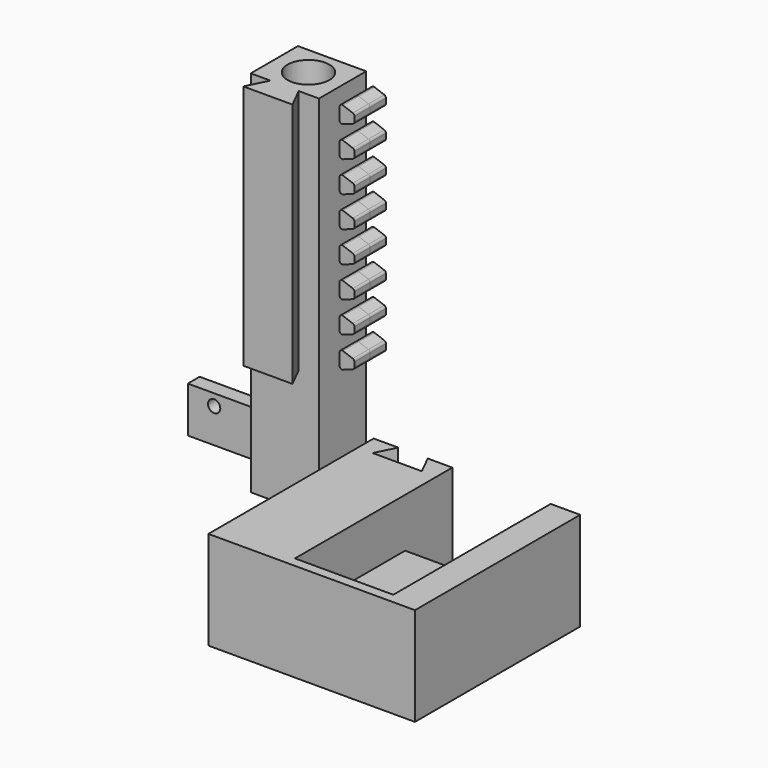
from build123d import *

# Parameters (mm, degrees)
F0_W      = 42
F0_H      = 42
F1_DEPTH  = 20
F3_DEPTH  = 20.001
F5_DEPTH  = 10
F6_W      = 7
F6_H      = 8
F7_DEPTH  = 10.001
F9_DEPTH  = 75
F11_D     = 8.5
F12_W     = 20
F12_H     = 12
F13_DEPTH = 25
F15_D     = 2.5
F15_DEPTH = 10
F15_TIP   = 0.7510757738
F18_DEPTH = 4
F19_DEPTH = 4.015
F20_R     = 0.5
F20_2_R   = 0.5
F20_3_R   = 0.5
F20_4_R   = 0.5
F20_5_R   = 0.5
F20_6_R   = 0.5
F20_7_R   = 0.5
F20_8_R   = 0.5
F20_9_R   = 0.5
F20_10_R  = 0.5
F20_11_R  = 0.5
F20_12_R  = 0.5
F20_13_R  = 0.5
F20_14_R  = 0.5
F20_15_R  = 0.5
F20_16_R  = 0.5
F21_R     = 1.5
F22_DEPTH = 2.02450667
F23_W     = 3
F23_H     = 9.305
F24_DEPTH = 20
F25_R     = 1.25
F26_DEPTH = 25
F27_W     = 14.144278072
F27_H     = 7.7009366201
F28_DEPTH = 25


# Not quite as in the source:
# - a feature names something its author has since deleted; it is built from what else it names


with BuildPart() as f1:
    # F0 (on Top) → F1 (new body)
    with BuildSketch(Plane.XY):
        with Locations((-0.6666667579, -21)):
            Rectangle(F0_W, F0_H)
    extrude(amount=F1_DEPTH)

    # F2 (on face) → F3 (cut, through all)
    with BuildSketch(Plane.XY.offset(20)):
        Polygon((-13.6666667579, 0), (-16.6666667579, 0), (-18.6666667579, -4), (-13.6666667579, -4), align=None)
        Polygon((-10.6666667579, 0), (-13.6666667579, 0), (-13.6666667579, -4), (-8.6666667579, -4), align=None)
    extrude(amount=-F3_DEPTH, mode=Mode.SUBTRACT)

    # F4 (on face) → F5 (cut)
    with BuildSketch(Plane.XY.offset(20)):
        Polygon((14.3333332421, 0), (0, 0), (-5.6666667579, 0), (-5.6666667579, -40), (14.3333332421, -40), align=None)
    extrude(amount=-F5_DEPTH, mode=Mode.SUBTRACT)

    # F6 (on face) → F7 (cut, through all)
    with BuildSketch(Plane.XY.offset(10)):
        with Locations((4.3333332421, -36)):
            Rectangle(F6_W, F6_H)
    extrude(amount=-F7_DEPTH, mode=Mode.SUBTRACT)

    # F12 (on face) → F13 (cut)
    with BuildSketch(Plane.XY.offset(10)):
        with Locations((4.3333332421, -6)):
            Rectangle(F12_W, F12_H)
    extrude(amount=-F13_DEPTH, mode=Mode.SUBTRACT)

    # F15
    with Locations(Plane(origin=(0, -12, 0), x_dir=(-1, 0, 0), z_dir=(0, 1, 0))):
        with Locations((-9.3333332421, 5.5), (0.6666667579, 5.5)):
            Hole(F15_D / 2, depth=F15_DEPTH)
            with Locations((0, 0, -(F15_DEPTH + F15_TIP / 2))):  # 118° drill point
                Cone(0, F15_D / 2, F15_TIP, mode=Mode.SUBTRACT)


with BuildPart() as f9:
    # F8 (on Top) → F9 (new body)
    with BuildSketch(Plane.XY):
        Polygon((-45.3414317595, 3.3614712143), (-45.4664317595, 3.1114712143), (-42.4664317595, 3.1114712143), (-42.4664317595, 15.3614712143), (-49.3414317595, 15.3614712143), (-49.3414317595, 3.3614712143), align=None)
        Polygon((-45.4664317595, 3.1114712143), (-47.4664317595, -0.8885287857), (-42.4664317595, -0.8885287857), (-42.4664317595, 3.1114712143), align=None)
        Polygon((-42.4664317595, 3.1114712143), (-42.4664317595, -0.8885287857), (-37.4664317595, -0.8885287857), (-39.4664317595, 3.1114712143), align=None)
        Polygon((-42.4664317595, 15.3614712143), (-42.4664317595, 3.1114712143), (-39.4664317595, 3.1114712143), (-39.5914317595, 3.3614712143), (-35.4664317595, 3.3614712143), (-35.4664317595, 15.3614712143), align=None)
    extrude(amount=F9_DEPTH)

    # F11 (through all)
    with Locations(Plane.XY.offset(75)):
        with Locations((-42.4039317595, 9.3614712143)):
            Hole(F11_D / 2)

    # F21 (on face) → F22 (cut, through all)
    with BuildSketch(Plane(origin=(0, 15.3614712143, 0), x_dir=(-1, 0, 0), z_dir=(0, 1, 0))):
        with Locations((42.4039317595, 68)):
            Circle(F21_R)
    extrude(amount=-F22_DEPTH, mode=Mode.SUBTRACT)

    # F23 (on face) → F24 (join)
    with BuildSketch(Plane(origin=(-49.3414317595, 0, 0), x_dir=(0, -1, 0), z_dir=(-1, 0, 0))):
        with Locations((-13.8614712143, 4.6525)):
            Rectangle(F23_W, F23_H)
    extrude(amount=F24_DEPTH)

    # F25 (on face) → F26 (cut)
    with BuildSketch(Plane(origin=(0, 15.3614712143, 0), x_dir=(-1, 0, 0), z_dir=(0, 1, 0))):
        with Locations((54.6914317595, 7)):
            Circle(F25_R)
        with Locations((63.9914317595, 7)):
            Circle(F25_R)
    extrude(amount=-F26_DEPTH, mode=Mode.SUBTRACT)

    # F27 (on face) → F28 (cut)
    with BuildSketch(Plane(origin=(0, 0, 0), x_dir=(1, 0, 0), z_dir=(0, 0, -1))):
        with Locations((-42.2692927235, 0.4889970957)):
            Rectangle(F27_W, F27_H)
    extrude(amount=-F28_DEPTH, mode=Mode.SUBTRACT)


with BuildPart() as f18:
    # F17 (on offset) → F18 (new body)
    with BuildSketch(Plane.XZ.offset(-11.3614712143)):
        Polygon((-34.4733819366, 69.08), (-31.4664317595, 70.1744403604), (-31.4664317595, 70.3041268816), (-31.4664317595, 71.8605594233), (-34.4733819366, 72.9549997837), align=None)
    extrude(amount=F18_DEPTH)

    # F20
    f20_edges = [f18.edges().sort_by_distance(p)[0] for p in [
        (-31.466432, 9.361471, 70.17444),
        (-31.466432, 9.361471, 71.860559),
        (-34.473382, 9.361471, 72.955),
        (-34.473382, 9.361471, 69.08),
    ]]
    fillet(f20_edges, radius=F20_R)


with BuildPart() as f18b:
    # F17 (on offset) → F18, piece 2 (new body)
    with BuildSketch(Plane.XZ.offset(-11.3614712143)):
        Polygon((-34.4733819366, 62.8), (-31.4664317595, 63.8944403604), (-31.4664317595, 64.0241268816), (-31.4664317595, 65.3069223761), (-31.4664317595, 65.5805594233), (-34.4733819366, 66.6749997837), align=None)
    extrude(amount=F18_DEPTH)

    # F20#2
    f20_2_edges = [f18b.edges().sort_by_distance(p)[0] for p in [
        (-34.473382, 9.361471, 62.8),
        (-31.466432, 9.361471, 63.89444),
        (-31.466432, 9.361471, 65.580559),
        (-34.473382, 9.361471, 66.675),
    ]]
    fillet(f20_2_edges, radius=F20_2_R)


with BuildPart() as f18c:
    # F17 (on offset) → F18, piece 3 (new body)
    with BuildSketch(Plane.XZ.offset(-11.3614712143)):
        Polygon((-34.4733819366, 56.52), (-31.4664317595, 57.6144403604), (-31.4664317595, 57.7441268816), (-31.4664317595, 59.0269223761), (-31.4664317595, 59.3005594233), (-34.4733819366, 60.3949997837), align=None)
    extrude(amount=F18_DEPTH)

    # F20#3
    f20_3_edges = [f18c.edges().sort_by_distance(p)[0] for p in [
        (-31.466432, 9.361471, 57.61444),
        (-34.473382, 9.361471, 56.52),
        (-31.466432, 9.361471, 59.300559),
        (-34.473382, 9.361471, 60.395),
    ]]
    fillet(f20_3_edges, radius=F20_3_R)


with BuildPart() as f18d:
    # F17 (on offset) → F18, piece 4 (new body)
    with BuildSketch(Plane.XZ.offset(-11.3614712143)):
        Polygon((-34.4733819366, 50.24), (-31.4664317595, 51.3344403604), (-31.4664317595, 51.4641268816), (-31.4664317595, 52.7469223761), (-31.4664317595, 53.0205594233), (-34.4733819366, 54.1149997837), align=None)
    extrude(amount=F18_DEPTH)

    # F20#4
    f20_4_edges = [f18d.edges().sort_by_distance(p)[0] for p in [
        (-34.473382, 9.361471, 50.24),
        (-31.466432, 9.361471, 51.33444),
        (-34.473382, 9.361471, 54.115),
        (-31.466432, 9.361471, 53.020559),
    ]]
    fillet(f20_4_edges, radius=F20_4_R)


with BuildPart() as f18e:
    # F17 (on offset) → F18, piece 5 (new body)
    with BuildSketch(Plane.XZ.offset(-11.3614712143)):
        Polygon((-34.4733819366, 43.96), (-31.4664317595, 45.0544403604), (-31.4664317595, 45.1841268816), (-31.4664317595, 46.4669223761), (-31.4664317595, 46.7405594233), (-34.4733819366, 47.8349997837), align=None)
    extrude(amount=F18_DEPTH)

    # F20#5
    f20_5_edges = [f18e.edges().sort_by_distance(p)[0] for p in [
        (-34.473382, 9.361471, 43.96),
        (-31.466432, 9.361471, 45.05444),
        (-31.466432, 9.361471, 46.740559),
        (-34.473382, 9.361471, 47.835),
    ]]
    fillet(f20_5_edges, radius=F20_5_R)


with BuildPart() as f18f:
    # F17 (on offset) → F18, piece 6 (new body)
    with BuildSketch(Plane.XZ.offset(-11.3614712143)):
        Polygon((-34.4733819366, 37.68), (-31.4664317595, 38.7744403604), (-31.4664317595, 38.9041268816), (-31.4664317595, 40.1869223761), (-31.4664317595, 40.4605594233), (-34.4733819366, 41.5549997837), align=None)
    extrude(amount=F18_DEPTH)

    # F20#6
    f20_6_edges = [f18f.edges().sort_by_distance(p)[0] for p in [
        (-31.466432, 9.361471, 38.77444),
        (-34.473382, 9.361471, 37.68),
        (-31.466432, 9.361471, 40.460559),
        (-34.473382, 9.361471, 41.555),
    ]]
    fillet(f20_6_edges, radius=F20_6_R)


with BuildPart() as f18g:
    # F17 (on offset) → F18, piece 7 (new body)
    with BuildSketch(Plane.XZ.offset(-11.3614712143)):
        Polygon((-34.4733819366, 31.4), (-31.4664317595, 32.4944403604), (-31.4664317595, 32.6241268816), (-31.4664317595, 33.9069223761), (-31.4664317595, 34.1805594233), (-34.4733819366, 35.2749997837), align=None)
    extrude(amount=F18_DEPTH)

    # F20#7
    f20_7_edges = [f18g.edges().sort_by_distance(p)[0] for p in [
        (-31.466432, 9.361471, 32.49444),
        (-34.473382, 9.361471, 31.4),
        (-31.466432, 9.361471, 34.180559),
        (-34.473382, 9.361471, 35.275),
    ]]
    fillet(f20_7_edges, radius=F20_7_R)


with BuildPart() as f18h:
    # F17 (on offset) → F18, piece 8 (new body)
    with BuildSketch(Plane.XZ.offset(-11.3614712143)):
        Polygon((-34.4733819366, 25.12), (-31.4664317595, 26.2144403604), (-31.4664317595, 26.3441268816), (-31.4664317595, 27.6269223761), (-31.4664317595, 27.9005594233), (-34.4733819366, 28.9949997837), align=None)
    extrude(amount=F18_DEPTH)

    # F20#8
    f20_8_edges = [f18h.edges().sort_by_distance(p)[0] for p in [
        (-31.466432, 9.361471, 26.21444),
        (-34.473382, 9.361471, 25.12),
        (-31.466432, 9.361471, 27.900559),
        (-34.473382, 9.361471, 28.995),
    ]]
    fillet(f20_8_edges, radius=F20_8_R)


with BuildPart() as f19:
    # F17 (on offset) → F19 (new body)
    with BuildSketch(Plane.XZ.offset(-11.3614712143)):
        Polygon((-34.4733819366, 37.68), (-31.4664317595, 38.7744403604), (-31.4664317595, 38.9041268816), (-31.4664317595, 40.1869223761), (-31.4664317595, 40.4605594233), (-34.4733819366, 41.5549997837), align=None)
    extrude(amount=-F19_DEPTH)

    # F20#9
    f20_9_edges = [f19.edges().sort_by_distance(p)[0] for p in [
        (-31.466432, 13.368971, 38.77444),
        (-34.473382, 13.368971, 37.68),
        (-31.466432, 13.368971, 40.460559),
        (-34.473382, 13.368971, 41.555),
    ]]
    fillet(f20_9_edges, radius=F20_9_R)


with BuildPart() as f19b:
    # F17 (on offset) → F19, piece 2 (new body)
    with BuildSketch(Plane.XZ.offset(-11.3614712143)):
        Polygon((-34.4733819366, 50.24), (-31.4664317595, 51.3344403604), (-31.4664317595, 51.4641268816), (-31.4664317595, 52.7469223761), (-31.4664317595, 53.0205594233), (-34.4733819366, 54.1149997837), align=None)
    extrude(amount=-F19_DEPTH)

    # F20#10
    f20_10_edges = [f19b.edges().sort_by_distance(p)[0] for p in [
        (-34.473382, 13.368971, 50.24),
        (-31.466432, 13.368971, 51.33444),
        (-34.473382, 13.368971, 54.115),
        (-31.466432, 13.368971, 53.020559),
    ]]
    fillet(f20_10_edges, radius=F20_10_R)


with BuildPart() as f19c:
    # F17 (on offset) → F19, piece 3 (new body)
    with BuildSketch(Plane.XZ.offset(-11.3614712143)):
        Polygon((-34.4733819366, 62.8), (-31.4664317595, 63.8944403604), (-31.4664317595, 64.0241268816), (-31.4664317595, 65.3069223761), (-31.4664317595, 65.5805594233), (-34.4733819366, 66.6749997837), align=None)
    extrude(amount=-F19_DEPTH)

    # F20#11
    f20_11_edges = [f19c.edges().sort_by_distance(p)[0] for p in [
        (-34.473382, 13.368971, 62.8),
        (-31.466432, 13.368971, 63.89444),
        (-31.466432, 13.368971, 65.580559),
        (-34.473382, 13.368971, 66.675),
    ]]
    fillet(f20_11_edges, radius=F20_11_R)


with BuildPart() as f19d:
    # F17 (on offset) → F19, piece 4 (new body)
    with BuildSketch(Plane.XZ.offset(-11.3614712143)):
        Polygon((-34.4733819366, 69.08), (-31.4664317595, 70.1744403604), (-31.4664317595, 70.3041268816), (-31.4664317595, 71.8605594233), (-34.4733819366, 72.9549997837), align=None)
    extrude(amount=-F19_DEPTH)

    # F20#12
    f20_12_edges = [f19d.edges().sort_by_distance(p)[0] for p in [
        (-31.466432, 13.368971, 70.17444),
        (-31.466432, 13.368971, 71.860559),
        (-34.473382, 13.368971, 72.955),
        (-34.473382, 13.368971, 69.08),
    ]]
    fillet(f20_12_edges, radius=F20_12_R)


with BuildPart() as f19e:
    # F17 (on offset) → F19, piece 5 (new body)
    with BuildSketch(Plane.XZ.offset(-11.3614712143)):
        Polygon((-34.4733819366, 25.12), (-31.4664317595, 26.2144403604), (-31.4664317595, 26.3441268816), (-31.4664317595, 27.6269223761), (-31.4664317595, 27.9005594233), (-34.4733819366, 28.9949997837), align=None)
    extrude(amount=-F19_DEPTH)

    # F20#13
    f20_13_edges = [f19e.edges().sort_by_distance(p)[0] for p in [
        (-34.473382, 13.368971, 25.12),
        (-31.466432, 13.368971, 26.21444),
        (-31.466432, 13.368971, 27.900559),
        (-34.473382, 13.368971, 28.995),
    ]]
    fillet(f20_13_edges, radius=F20_13_R)


with BuildPart() as f19f:
    # F17 (on offset) → F19, piece 6 (new body)
    with BuildSketch(Plane.XZ.offset(-11.3614712143)):
        Polygon((-34.4733819366, 31.4), (-31.4664317595, 32.4944403604), (-31.4664317595, 32.6241268816), (-31.4664317595, 33.9069223761), (-31.4664317595, 34.1805594233), (-34.4733819366, 35.2749997837), align=None)
    extrude(amount=-F19_DEPTH)

    # F20#14
    f20_14_edges = [f19f.edges().sort_by_distance(p)[0] for p in [
        (-31.466432, 13.368971, 32.49444),
        (-34.473382, 13.368971, 31.4),
        (-31.466432, 13.368971, 34.180559),
        (-34.473382, 13.368971, 35.275),
    ]]
    fillet(f20_14_edges, radius=F20_14_R)


with BuildPart() as f19g:
    # F17 (on offset) → F19, piece 7 (new body)
    with BuildSketch(Plane.XZ.offset(-11.3614712143)):
        Polygon((-34.4733819366, 43.96), (-31.4664317595, 45.0544403604), (-31.4664317595, 45.1841268816), (-31.4664317595, 46.4669223761), (-31.4664317595, 46.7405594233), (-34.4733819366, 47.8349997837), align=None)
    extrude(amount=-F19_DEPTH)

    # F20#15
    f20_15_edges = [f19g.edges().sort_by_distance(p)[0] for p in [
        (-34.473382, 13.368971, 43.96),
        (-31.466432, 13.368971, 45.05444),
        (-31.466432, 13.368971, 46.740559),
        (-34.473382, 13.368971, 47.835),
    ]]
    fillet(f20_15_edges, radius=F20_15_R)


with BuildPart() as f19h:
    # F17 (on offset) → F19, piece 8 (new body)
    with BuildSketch(Plane.XZ.offset(-11.3614712143)):
        Polygon((-34.4733819366, 56.52), (-31.4664317595, 57.6144403604), (-31.4664317595, 57.7441268816), (-31.4664317595, 59.0269223761), (-31.4664317595, 59.3005594233), (-34.4733819366, 60.3949997837), align=None)
    extrude(amount=-F19_DEPTH)

    # F20#16
    f20_16_edges = [f19h.edges().sort_by_distance(p)[0] for p in [
        (-31.466432, 13.368971, 57.61444),
        (-34.473382, 13.368971, 56.52),
        (-31.466432, 13.368971, 59.300559),
        (-34.473382, 13.368971, 60.395),
    ]]
    fillet(f20_16_edges, radius=F20_16_R)


solid = Compound([f1.part, f9.part, f18.part, f18b.part, f18c.part, f18d.part, f18e.part, f18f.part, f18g.part, f18h.part, f19.part, f19b.part, f19c.part, f19d.part, f19e.part, f19f.part, f19g.part, f19h.part])
